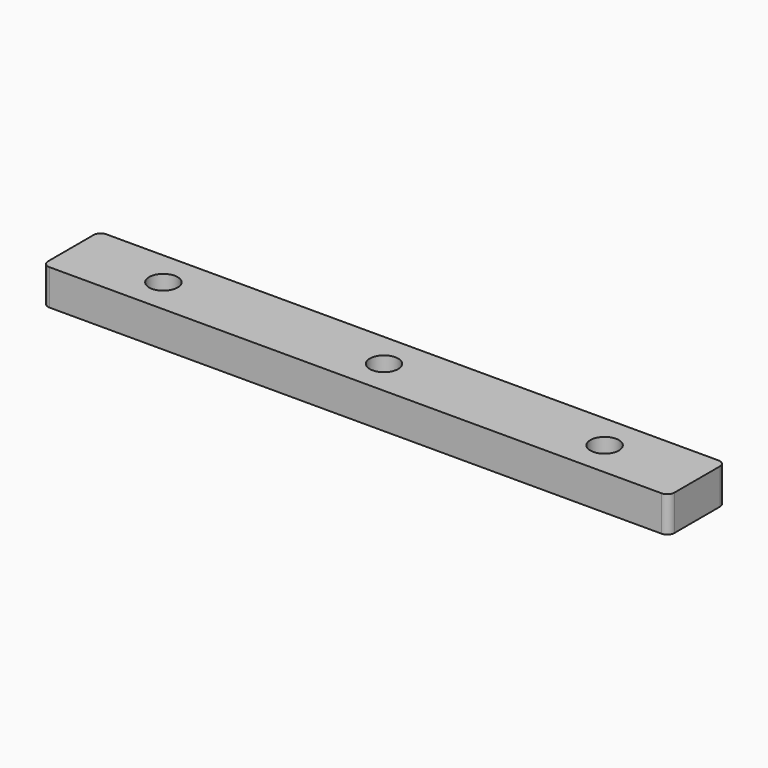
from build123d import *

# Parameters (mm, degrees)
F0_W     = 440
F0_H     = 50
F0_R     = 10
F1_DEPTH = 25
F2_R     = 5


# Not quite as in the source:
# - a feature of the source that left no trace in its solid (it failed there, or was rolled back) is left out


with BuildPart() as f1:
    # F0 (on Top) → F1 (new body)
    with BuildSketch(Plane.XY):
        Rectangle(F0_W, F0_H)
        with Locations((-155, 0)):
            Circle(F0_R, mode=Mode.SUBTRACT)
        Circle(F0_R, mode=Mode.SUBTRACT)
        with Locations((155, 0)):
            Circle(F0_R, mode=Mode.SUBTRACT)
    extrude(amount=F1_DEPTH)

    # F2
    f2_edges = [f1.edges().sort_by_distance(p)[0] for p in [
        (-220, -25, 12.5),
        (220, -25, 12.5),
        (220, 25, 12.5),
        (-220, 25, 12.5),
    ]]
    fillet(f2_edges, radius=F2_R)


solid = f1.part
